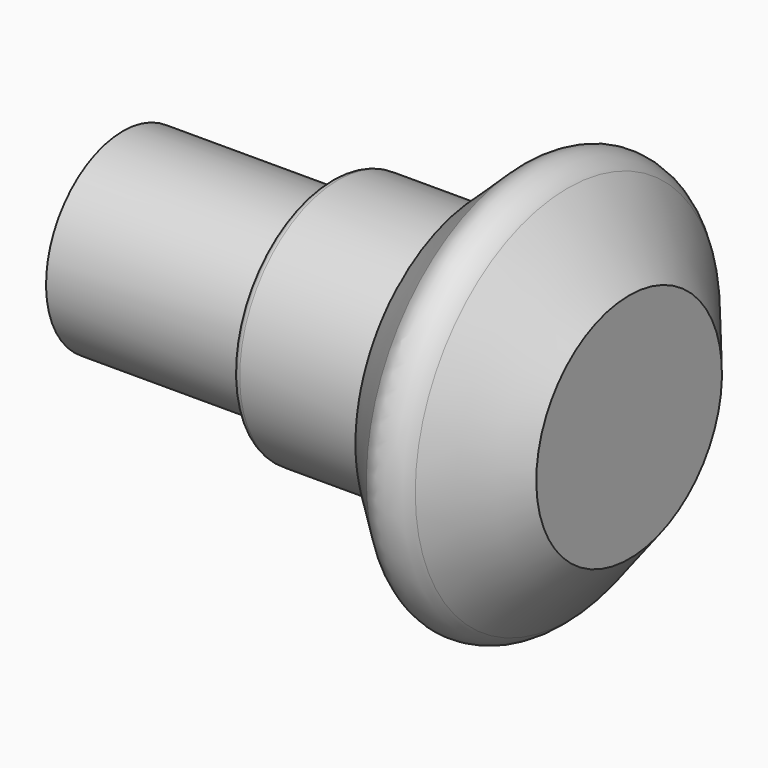
from build123d import *


with BuildPart() as f1:
    # F0 (on Front) → F1 (revolve)
    with BuildSketch(Plane.XZ):
        with BuildLine():
            Line((0, 15.100086289), (-7.9947902337, 24.7891377658))
            add(Edge.make_bspline(
                [(-13.5336209388, 25.8130880211), (-13.1794829922, 26.0396653478), (-12.3469790571, 26.5077257402), (-10.9534140953, 26.5328921513), (-9.365299038, 26.0844114305), (-8.2402056984, 25.1083988869), (-8.0565123354, 24.8694320839), (-7.9947902337, 24.7891377658)],
                knots=[0.0753740232, 0.0753740232, 0.0753740232, 0.0753740232, 0.236653892, 0.4524170896, 0.6819552068, 0.89313499, 1, 1, 1, 1], degree=3))
            Line((-13.5336209388, 25.8130880211), (-19.239403379, 20.4293505417))
            ThreePointArc((-19.239403379, 20.4293505417), (-19.7032923995, 19.7667886958), (-19.8668379088, 18.9746813235))
            Line((-19.8668379088, 18.9746813235), (-19.8668367383, 17.0000005928))
            ThreePointArc((-19.8668367383, 17.0000005928), (-20.1597297475, 16.2928934284), (-20.8668367383, 16))
            Line((-20.8668367383, 16), (-37.8668361455, 16))
            ThreePointArc((-37.8668361455, 16), (-38.5739429267, 15.7071067812), (-38.8668361455, 15))
            Line((-38.8668361455, 15), (-38.8668361455, 13.5))
            ThreePointArc((-38.8668361455, 13.5), (-39.1597293643, 12.7928932188), (-39.8668361455, 12.5))
            Line((-39.8668361455, 12.5), (-65.8668361455, 12.5))
            Line((-65.8668361455, 12.5), (-65.8668361455, 0))
            Line((-65.8668361455, 0), (-26.8668361455, 0))
            Line((-26.8668361455, 0), (-19.8668361455, 0))
            Line((-19.8668361455, 0), (0, 0))
            Line((0, 0), (0, 15.100086289))
        make_face()
    revolve(axis=Axis((-46.3668361455, 0, 0), (-1, 0, 0)))


solid = f1.part
